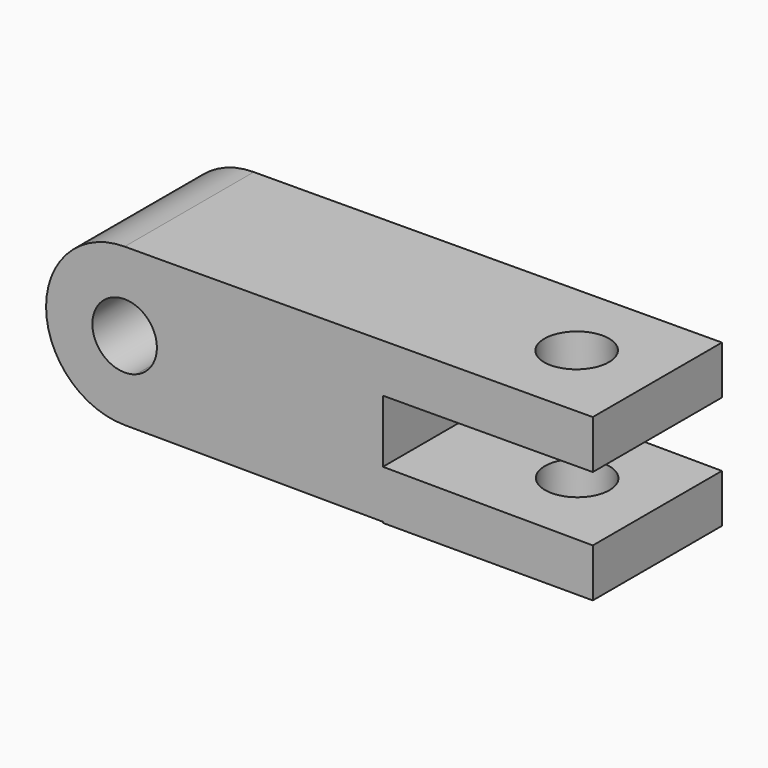
from build123d import *

# Parameters (mm, degrees)
F0_W     = 107.95
F0_H     = 31.75
F1_DEPTH = 31.75
F3_DEPTH = 31.751
F5_DEPTH = 31.7506558501


with BuildPart() as f1:
    # F0 (on Front) → F1 (new body)
    with BuildSketch(Plane.XZ):
        with Locations((1.144817099, -4.4740095741)):
            Rectangle(F0_W, F0_H)
    extrude(amount=F1_DEPTH)

    # F2 (on face) → F3 (cut, through all)
    with BuildSketch(Plane.XZ.offset(31.75)):
        with BuildLine():
            ThreePointArc((-34.6886992289, -10.405750614), (-31.724758859, -8.0747267722), (-30.605182901, -4.4740095741))
            ThreePointArc((-30.605182901, -4.4740095741), (-31.724758859, -0.8732923759), (-34.6886992289, 1.4577314658))
            ThreePointArc((-34.6886992289, 1.4577314658), (-43.305182901, -4.4740095741), (-34.6886992289, -10.405750614))
        make_face()
        with BuildLine():
            ThreePointArc((-36.955182901, -19.9203009288), (-52.4014742558, -4.4740095741), (-36.955182901, 10.9722817806))
            Line((-36.955182901, 10.9722817806), (55.119817099, 11.4009904259))
            Line((55.119817099, 11.4009904259), (-52.830182901, 11.4009904259))
            Line((-52.830182901, 11.4009904259), (-52.830182901, -20.3490095741))
            Line((-52.830182901, -20.3490095741), (13.844817099, -20.3490095741))
            Line((13.844817099, -20.3490095741), (13.844817099, -20.1568298366))
            Line((13.844817099, -20.1568298366), (-36.955182901, -19.9203009288))
        make_face()
        Polygon((55.119817099, -10.823906328), (55.119817099, 1.8758871798), (13.844817099, 1.6837074423), (13.844817099, -10.6317265905), align=None)
    extrude(amount=-F3_DEPTH, mode=Mode.SUBTRACT)

    # F4 (on face) → F5 (cut, through all)
    with BuildSketch(Plane(origin=(-0.051887861, 0, 11.1441065064), x_dir=(0.9999891606, 0, 0.0046560304), z_dir=(-0.0046560304, 0, 0.9999891606))):
        with BuildLine():
            ThreePointArc((38.2637782771, -22.1403273388), (43.4058074687, -20.7167652744), (45.6473029929, -15.875))
            ThreePointArc((45.6473029929, -15.875), (35.1887985171, -11.0332347256), (38.2637782771, -22.1403273388))
        make_face()
    extrude(amount=-F5_DEPTH, mode=Mode.SUBTRACT)


solid = f1.part
